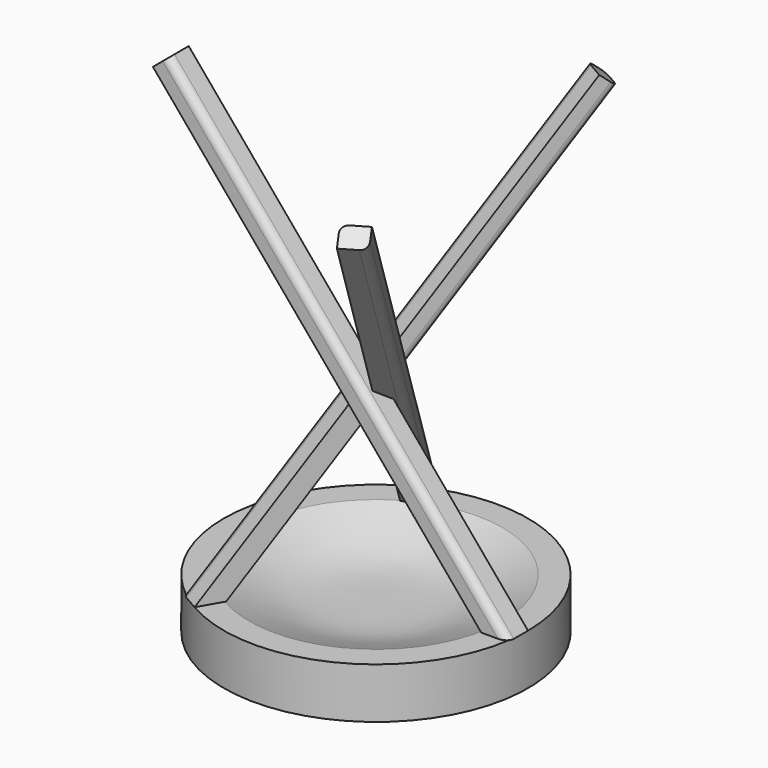
from build123d import *

# Parameters (mm, degrees)
F0_W         = 5
F0_H         = 10
F3_DEPTH     = 5
F4_COUNT     = 3
F5_T4_DEPTH  = 64.961938704
F5_T9_DEPTH  = 108.2772549851
F5_T14_DEPTH = 111.6336535099
F5_T19_DEPTH = 111.6336535099
F5_T24_DEPTH = 64.3133444777
F5_T29_DEPTH = 64.3133444777
F5_T34_DEPTH = 108.2772549851


# Not quite as in the source:
# - a fillet or chamfer that OpenCascade refuses, or shapes differently, is made with other operations: its cross-section is extruded or revolved along the edge and cut away or added


with BuildPart() as f1:
    # F0 (on Front) → F1 (revolve)
    with BuildSketch(Plane.XZ):
        with Locations((-27.5, 5)):
            Rectangle(F0_W, F0_H)
        with BuildLine():
            Line((-25, 10), (-25, 0))
            Line((-25, 0), (0, 0))
            Line((0, 0), (0, 5))
            add(Edge.make_bspline(
                [(-25, 10), (-12.5, 5), (-12.5, 5), (0, 5)],
                knots=[0, 0, 0, 0, 25.495097568, 25.495097568, 25.495097568, 25.495097568], degree=3))
        make_face()
    revolve(axis=Axis((0, 0, 2.5), (0, 0, -1)))

    # F2 (on Front) → F3 (join)
    with BuildSketch(Plane.XZ):
        Polygon((24.7783708427, 10), (30, 10), (-36.9358222275, 89.7710066129), (-40, 87.1998561742), align=None)
    extrude(amount=F3_DEPTH)

    # F4: F1 ×3 about axis
    f4_axis = Axis((0, 0, 2.5), (0, 0, -1))


with BuildPart() as f1_1:
    add(f1.part)
    for i in range(1, F4_COUNT):
        add(f1.part.rotate(f4_axis, i * 360 / F4_COUNT))

    # F5: fillet of radius 1.5 on 7 edges, made by hand


with BuildPart() as f5_tool2:
    # F5_s3 → F5_t4 (new body)
    with BuildSketch(Plane(origin=(10.0591539469, -17.4229657171, 23.9760657093), x_dir=(0.8660254038, 0.5, 0), z_dir=(0.3213938048, -0.5566703992, 0.7660444431))):
        with BuildLine():
            ThreePointArc((1.5, 29.4092093904), (0.4393398282, 28.9698695622), (0, 27.9092093904))
            Line((0, 27.9092093904), (0, 29.4092093904))
            Line((0, 29.4092093904), (1.5, 29.4092093904))
        make_face()
    extrude(amount=F5_T4_DEPTH)

    split(bisect_by=Plane(origin=(22.5287614301, 0, 18.9038754068), x_dir=(0, 1, 0), z_dir=(0.7660444431, 0, 0.6427876097)), keep=Keep.TOP)


with BuildPart() as f1_2:
    add(f1_1.part)

    # F5_t1: cut F5_tool2
    add(f5_tool2.part, mode=Mode.SUBTRACT)


with BuildPart() as f5_tool7:
    # F5_s8 → F5_t9 (new body)
    with BuildSketch(Plane(origin=(30.937518597, -53.58535407, 73.7397978677), x_dir=(-0.8660254038, -0.5, 0), z_dir=(-0.3213938048, 0.5566703992, -0.7660444431))):
        with BuildLine():
            ThreePointArc((-5, 26.9092093904), (-4.5606601718, 25.8485492187), (-3.5, 25.4092093904))
            Line((-3.5, 25.4092093904), (-5, 25.4092093904))
            Line((-5, 25.4092093904), (-5, 26.9092093904))
        make_face()
    extrude(amount=F5_T9_DEPTH)

    split(bisect_by=Plane.XY.offset(10), keep=Keep.TOP)


with BuildPart() as f1_3:
    add(f1_2.part)

    # F5_t6: cut F5_tool7
    add(f5_tool7.part, mode=Mode.SUBTRACT)


with BuildPart() as f5_tool12:
    # F5_s13 → F5_t14 (new body)
    with BuildSketch(Plane(origin=(9.8816921063, 0, -11.7765420685), x_dir=(0, 1, 0), z_dir=(-0.6427876097, 0, 0.7660444431))):
        with BuildLine():
            ThreePointArc((-5, -27.9092093904), (-4.5606601718, -28.9698695622), (-3.5, -29.4092093904))
            Line((-3.5, -29.4092093904), (-5, -29.4092093904))
            Line((-5, -29.4092093904), (-5, -27.9092093904))
        make_face()
    extrude(amount=F5_T14_DEPTH)

    split(bisect_by=Plane.XY.offset(10), keep=Keep.TOP)


with BuildPart() as f1_4:
    add(f1_3.part)

    # F5_t11: cut F5_tool12
    add(f5_tool12.part, mode=Mode.SUBTRACT)


with BuildPart() as f5_tool17:
    # F5_s18 → F5_t19 (new body)
    with BuildSketch(Plane(origin=(-4.9408460531, -8.5577963964, -11.7765420685), x_dir=(-0.8660254038, 0.5, 0), z_dir=(0.3213938048, 0.5566703992, 0.7660444431))):
        with BuildLine():
            ThreePointArc((5, 27.9092093904), (4.5606601718, 28.9698695622), (3.5, 29.4092093904))
            Line((3.5, 29.4092093904), (5, 29.4092093904))
            Line((5, 29.4092093904), (5, 27.9092093904))
        make_face()
    extrude(amount=F5_T19_DEPTH)

    split(bisect_by=Plane.XY.offset(10), keep=Keep.TOP)


with BuildPart() as f1_5:
    add(f1_4.part)

    # F5_t16: cut F5_tool17
    add(f5_tool17.part, mode=Mode.SUBTRACT)


with BuildPart() as f5_tool22:
    # F5_s23 → F5_t24 (new body)
    with BuildSketch(Plane(origin=(-61.8750371939, 0, 73.7397978677), x_dir=(0, 1, 0), z_dir=(0.6427876097, 0, -0.7660444431))):
        with BuildLine():
            ThreePointArc((-1.5, 25.4092093904), (-0.4393398282, 25.8485492187), (0, 26.9092093904))
            Line((0, 26.9092093904), (0, 25.4092093904))
            Line((0, 25.4092093904), (-1.5, 25.4092093904))
        make_face()
    extrude(amount=F5_T24_DEPTH)

    split(bisect_by=Plane(origin=(-11.264380715, -19.5104797142, 18.9038754068), x_dir=(0.8660254038, -0.5, 0), z_dir=(-0.3830222216, -0.6634139482, 0.6427876097)), keep=Keep.TOP)


with BuildPart() as f1_6:
    add(f1_5.part)

    # F5_t21: cut F5_tool22
    add(f5_tool22.part, mode=Mode.SUBTRACT)


with BuildPart() as f5_tool27:
    # F5_s28 → F5_t29 (new body)
    with BuildSketch(Plane(origin=(30.937518597, 53.58535407, 73.7397978677), x_dir=(0.8660254038, -0.5, 0), z_dir=(-0.3213938048, -0.5566703992, -0.7660444431))):
        with BuildLine():
            ThreePointArc((0, 26.9092093904), (-0.4393398282, 25.8485492187), (-1.5, 25.4092093904))
            Line((-1.5, 25.4092093904), (0, 25.4092093904))
            Line((0, 25.4092093904), (0, 26.9092093904))
        make_face()
    extrude(amount=F5_T29_DEPTH)

    split(bisect_by=Plane(origin=(-11.264380715, 19.5104797142, 18.9038754068), x_dir=(-0.8660254038, -0.5, 0), z_dir=(-0.3830222216, 0.6634139482, 0.6427876097)), keep=Keep.TOP)


with BuildPart() as f1_7:
    add(f1_6.part)

    # F5_t26: cut F5_tool27
    add(f5_tool27.part, mode=Mode.SUBTRACT)


with BuildPart() as f5_tool32:
    # F5_s33 → F5_t34 (new body)
    with BuildSketch(Plane(origin=(30.937518597, 53.58535407, 73.7397978677), x_dir=(0.8660254038, -0.5, 0), z_dir=(-0.3213938048, -0.5566703992, -0.7660444431))):
        with BuildLine():
            ThreePointArc((-5, 26.9092093904), (-4.5606601718, 25.8485492187), (-3.5, 25.4092093904))
            Line((-3.5, 25.4092093904), (-5, 25.4092093904))
            Line((-5, 25.4092093904), (-5, 26.9092093904))
        make_face()
    extrude(amount=F5_T34_DEPTH)

    split(bisect_by=Plane.XY.offset(10), keep=Keep.TOP)


with BuildPart() as f1_8:
    add(f1_7.part)

    # F5_t31: cut F5_tool32
    add(f5_tool32.part, mode=Mode.SUBTRACT)


solid = f1_8.part
